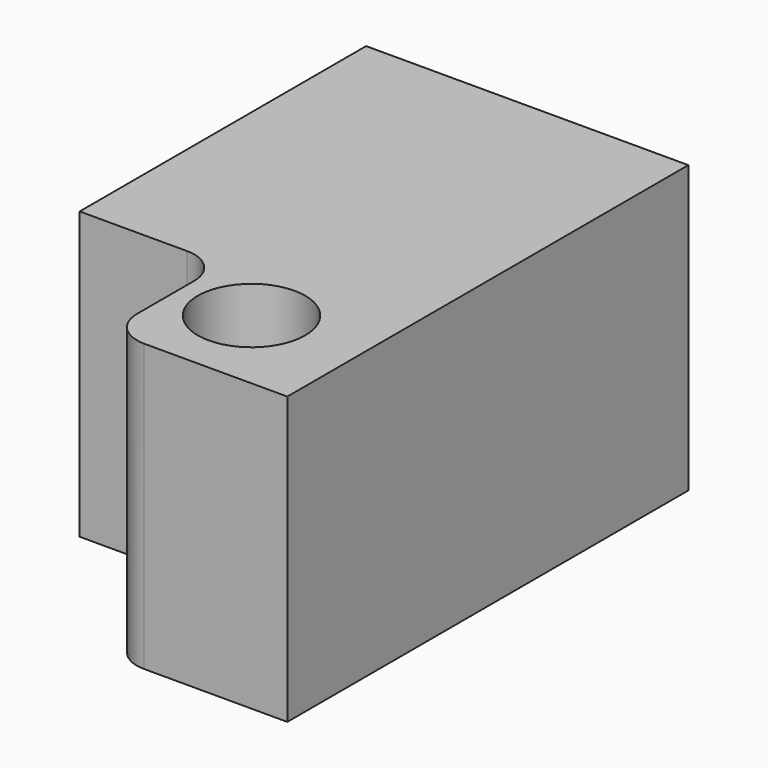
from build123d import *

# Parameters (mm, degrees)
F0_R     = 7.5
F1_DEPTH = 40


# Not quite as in the source:
# - a feature names something its author has since deleted; it is built from what else it names


with BuildPart() as f1:
    # F0 (on Top) → F1 (new body)
    with BuildSketch(Plane.XY):
        with BuildLine():
            Line((40, 0), (0, 0))
            Line((0, 0), (0, -5))
            Line((0, -5), (15, -5))
            ThreePointArc((15, -5), (18.5355339059, -6.4644660941), (20, -10))
            Line((20, -10), (20, -20))
            ThreePointArc((20, -20), (21.4644660941, -23.5355339059), (25, -25))
            Line((25, -25), (35, -25))
            Line((35, -25), (45, -25))
            Line((45, -25), (45, -19.1631559283))
            Line((45, -19.1631559283), (45, 0))
            Line((45, 0), (40, 0))
        make_face()
        with Locations((30, -12.5)):
            Circle(F0_R, mode=Mode.SUBTRACT)
        Polygon((0, 45), (0, 0), (40, 0), (45, 0), (45, 45), align=None)
    extrude(amount=F1_DEPTH)


solid = f1.part
